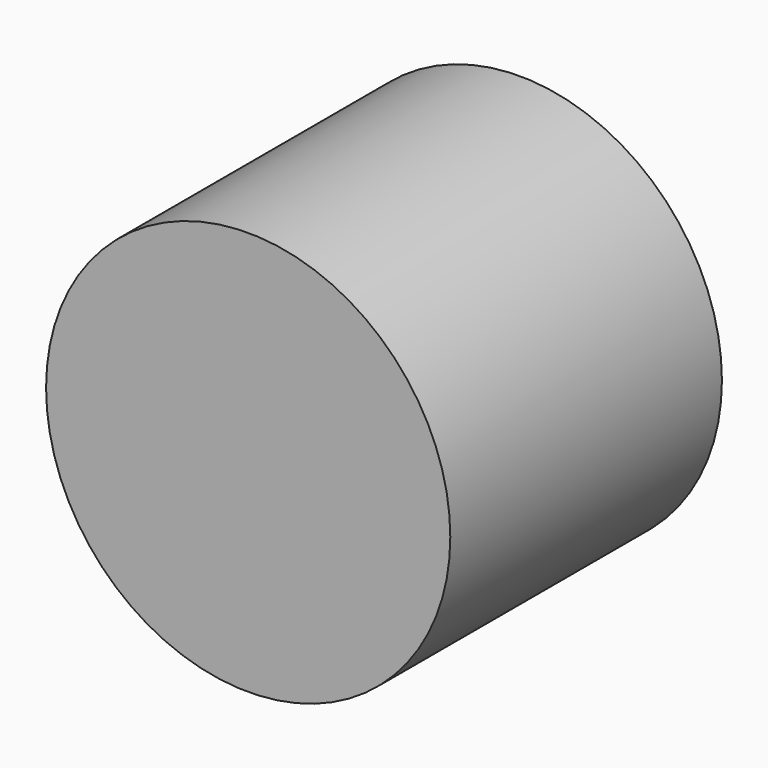
from build123d import *

# Parameters (mm, degrees)
F0_R     = 7.1063486515
F1_DEPTH = 11.938


# Not quite as in the source:
# - the program builds the solid bodies; features that only make, move or delete a surface that nothing else refers to are left out


with BuildPart() as f1:
    # F0 (on Front) → F1 (new body)
    with BuildSketch(Plane.XZ):
        with Locations((-66.341355443, 47.7696508169)):
            Circle(F0_R)
    extrude(amount=F1_DEPTH)


solid = f1.part
